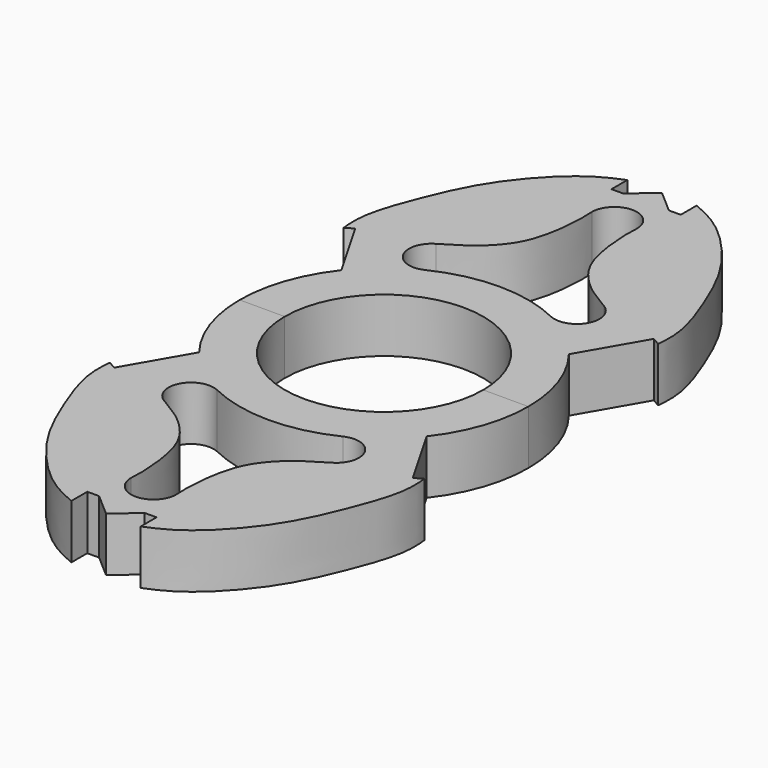
from build123d import *
from build123d import SkipClean  # not in build123d's __all__

# Parameters (mm, degrees)
F1_DEPTH = 6


# Not quite as in the source:
# - a pattern or mirror of a feature is missing from the dataset's text; its kind, count and spacing are read off the source's solid


with BuildPart() as f1:
    # F0 (on Top) → F1 (new body)
    with BuildSketch(Plane.XY):
        with BuildLine():
            Line((11, 0), (16, 0))
            ThreePointArc((16, 0), (15.1274260959, 5.2116196823), (12.6048775359, 9.854798948))
            ThreePointArc((12.6048775359, 9.854798948), (12.6039156913, 9.856029081), (12.6029537267, 9.8572591203))
            Line((12.6029537267, 9.8572591203), (16.5472631752, 16.6890034859))
            Line((16.5472631752, 16.6890034859), (17.413288579, 16.1890034859))
            add(Edge.make_bspline(
                [(17.413288579, 16.1890034859), (17.5041916061, 16.8045773234), (17.7045445822, 19.4085508868), (15.5298067399, 25.2595570372), (12.9266999082, 31.0960374777), (7.9390301641, 36.5896284217), (5.2735054472, 37.9125925094), (3.8379400503, 38.5036543012)],
                knots=[0, 0, 0, 0, 0.1468390725, 0.3630340887, 0.5865738984, 0.8170443021, 1, 1, 1, 1], degree=3))
            Line((3.8379400503, 38.5036543012), (3.8379400503, 36.3024744126))
            Line((3.8379400503, 36.3024744126), (2.5230119528, 36.3024744126))
            Line((2.5230119528, 36.3024744126), (0, 38.5036543012))
            Line((0, 38.5036543012), (-2.5230119528, 36.3024744126))
            Line((-2.5230119528, 36.3024744126), (-3.8379400503, 36.3024744126))
            Line((-3.8379400503, 36.3024744126), (-3.8379400503, 38.5036543012))
            add(Edge.make_bspline(
                [(-17.413288579, 16.1890034859), (-17.5041916061, 16.8045773234), (-17.7045445822, 19.4085508868), (-15.5298067399, 25.2595570372), (-12.9266999082, 31.0960374777), (-7.9390301641, 36.5896284217), (-5.2735054472, 37.9125925094), (-3.8379400503, 38.5036543012)],
                knots=[0, 0, 0, 0, 0.1468390725, 0.3630340887, 0.5865738984, 0.8170443021, 1, 1, 1, 1], degree=3))
            Line((-17.413288579, 16.1890034859), (-16.5472631752, 16.6890034859))
            Line((-16.5472631752, 16.6890034859), (-12.6029537267, 9.8572591203))
            ThreePointArc((-12.6029537267, 9.8572591203), (-12.6039156913, 9.856029081), (-12.6048775359, 9.854798948))
            ThreePointArc((-12.6048775359, 9.854798948), (-15.1274260959, 5.2116196823), (-16, 0))
            Line((-16, 0), (-11, 0))
            ThreePointArc((-11, 0), (0, 11), (11, 0))
        make_face()
        with BuildLine():
            ThreePointArc((-2.5, 31.9088473916), (0, 34.4088473916), (2.5, 31.9088473916))
            add(Edge.make_bspline(
                [(2.5, 31.9088473916), (2.4331220889, 30.6490394363), (2.4535157828, 30.0127263526), (2.8986373466, 23.7894092903), (6.9226723271, 20.1849518953), (7.2970524444, 20.0978087891), (9.3067939396, 18.8178154736)],
                knots=[0, 0, 0, 0, 0.191959096, 0.4953854958, 0.7661719362, 1, 1, 1, 1], degree=3))
            ThreePointArc((9.3067939396, 18.8178154736), (10.2567995477, 15.4836064725), (6.9615764655, 14.4061255414))
            ThreePointArc((6.9615764655, 14.4061255414), (0, 16), (-6.9615764655, 14.4061255414))
            ThreePointArc((-6.9615764655, 14.4061255414), (-10.2567995477, 15.4836064725), (-9.3067939396, 18.8178154736))
            add(Edge.make_bspline(
                [(-2.5, 31.9088473916), (-2.4331220889, 30.6490394363), (-2.4535157828, 30.0127263526), (-2.8986373466, 23.7894092903), (-6.9226723271, 20.1849518953), (-7.2970524444, 20.0978087891), (-9.3067939396, 18.8178154736)],
                knots=[0, 0, 0, 0, 0.191959096, 0.4953854958, 0.7661719362, 1, 1, 1, 1], degree=3))
        make_face(mode=Mode.SUBTRACT)
    extrude(amount=F1_DEPTH)

    # F1_copies: F1 across plane


with BuildPart() as f1_1:
    add(f1.part, clean=False)
    with SkipClean():  # cleaning this boolean's faces spoils the solid; the shape is the same uncleaned
        add(f1.part.mirror(Plane(origin=(0, 0, 0), x_dir=(0, 0, -1), z_dir=(0, -1, 0))), clean=False)


solid = f1_1.part
